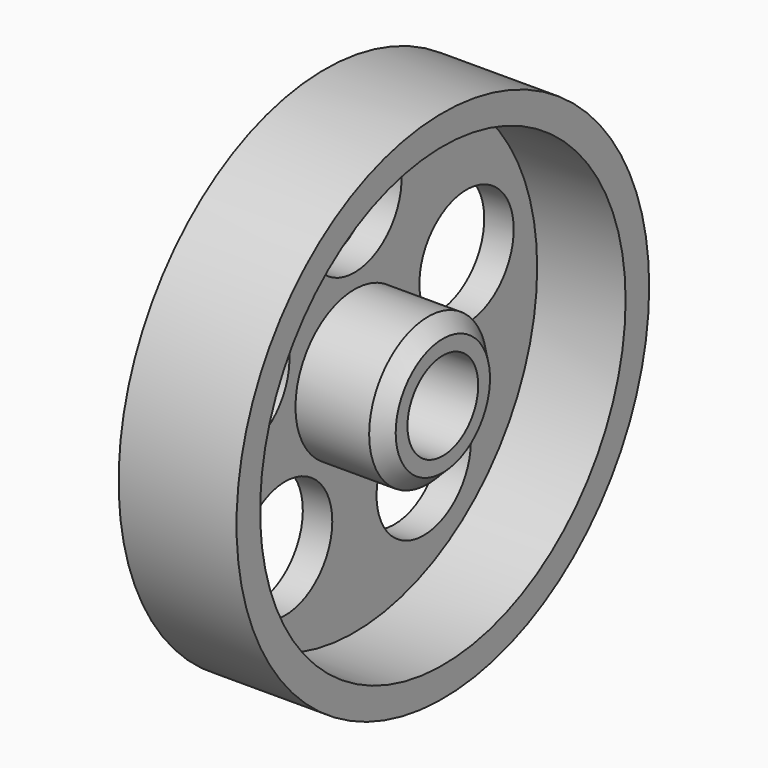
from build123d import *

# Parameters (mm, degrees)
F0_W            = 8
F0_H            = 17.5
F3_D            = 6
F4_T            = -2
F6_D            = 8
F6_COPIES_COUNT = 5
F7_SIZE         = 1


# Not quite as in the source:
# - a pattern or mirror of a feature is missing from the dataset's text; its kind, count and spacing are read off the source's solid


with BuildPart() as f1:
    # F0 (on Top) → F1 (revolve)
    with BuildSketch(Plane.XY):
        with Locations((4, 8.75)):
            Rectangle(F0_W, F0_H)
    revolve(axis=Axis((4, 0, 0), (1, 0, 0)))

    # F3 (through all)
    with Locations(Plane(origin=(0, 0, 0), x_dir=(0, 1, 0), z_dir=(-1, 0, 0))):
        with Locations((0, 0)):
            Hole(F3_D / 2)

    # F4
    f4_openings = [f1.faces().sort_by_distance(p)[0] for p in [
        (8, -17.005025, 0),
    ]]
    offset(amount=F4_T, openings=f4_openings)

    # F6 (through all)
    with Locations(Plane(origin=(0, 0, 0), x_dir=(0, 1, 0), z_dir=(-1, 0, 0))):
        with Locations((0, -10)):
            f6 = Hole(F6_D / 2)

    # F6_copies: F6 ×5 about axis
    f6_copies_axis = Axis((0, 0, 0), (1, 0, 0))
    for i in range(1, F6_COPIES_COUNT):
        add(f6.rotate(f6_copies_axis, i * 360 / F6_COPIES_COUNT), mode=Mode.SUBTRACT)

    # F7
    f7_edges = [f1.edges().sort_by_distance(p)[0] for p in [
        (8, -5, 0),
    ]]
    chamfer(f7_edges, length=F7_SIZE)


solid = f1.part
